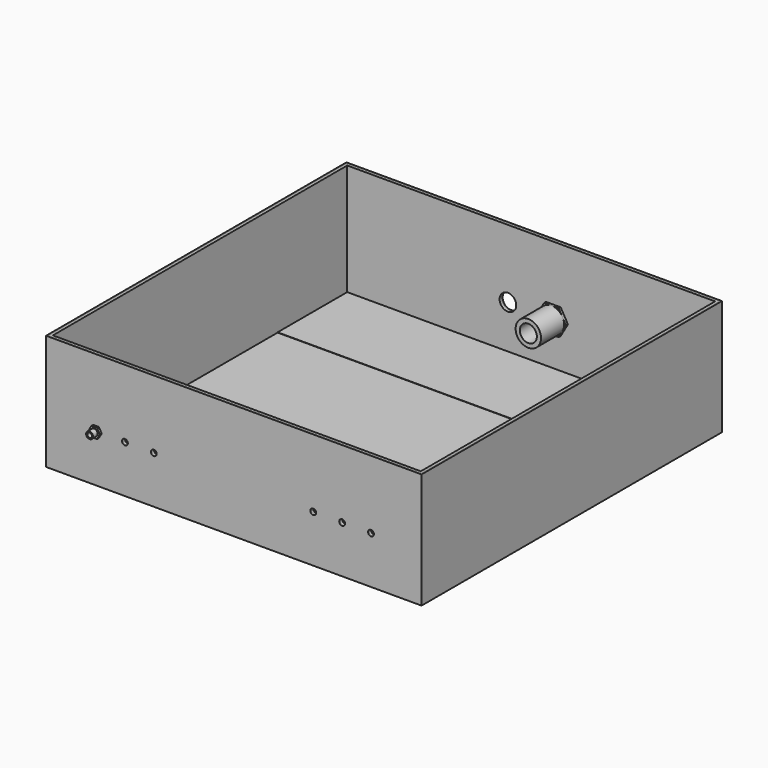
from build123d import *

# Parameters (mm, degrees)
F0_W      = 650
F0_H      = 650
F1_DEPTH  = 200
F2_T      = -2.5
F3_DEPTH  = 197.5
F4_T      = -4
F5_W      = 637
F5_H      = 150.622
F6_DEPTH  = 0.5
F7_R      = 5
F8_DEPTH  = 25
F9_R      = 14.3895
F10_DEPTH = 15
F11_R     = 4
F12_DEPTH = 4
F13_R     = 6
F13_R_2   = 4
F14_DEPTH = 10
F15_R     = 5
F15_R_2   = 4
F16_DEPTH = 6.5
F17_R     = 5
F17_R_2   = 4
F18_DEPTH = 4
F19_R     = 6
F19_R_2   = 5
F20_DEPTH = 150
F21_R     = 11.3895
F22_DEPTH = 4
F23_R     = 13.0309314184
F23_R_2   = 11.3895
F24_DEPTH = 25
F25_R     = 14.3895
F25_R_2   = 11.3895
F26_DEPTH = 6.5
F27_R     = 11.3895
F28_DEPTH = 4
F29_R     = 22.0019443752
F29_R_2   = 14.7554030698
F30_DEPTH = 50


# Not quite as in the source:
# - a feature names something its author has since deleted; it is built from what else it names


with BuildPart() as f1:
    # F0 (on Top) → F1 (new body)
    with BuildSketch(Plane.XY):
        Rectangle(F0_W, F0_H)
    extrude(amount=F1_DEPTH)

    # F2
    f2_openings = [f1.faces().sort_by_distance(p)[0] for p in [
        (0, 0, 200),
    ]]
    offset(amount=F2_T, openings=f2_openings)


with BuildPart() as f3:
    # F3 (new): a face of the model
    f3_faces = [f1.part.faces().sort_by_distance(p)[0] for p in [
        (0, 0, 2.5),
    ]]
    extrude(f3_faces, amount=F3_DEPTH)

    # F4
    f4_openings = [f3.faces().sort_by_distance(p)[0] for p in [
        (0, 0, 200),
    ]]
    offset(amount=F4_T, openings=f4_openings)

    # F5 (on face) → F6 (join)
    with BuildSketch(Plane.XY.offset(6.5)):
        with Locations((0, 243.189)):
            Rectangle(F5_W, F5_H)
    extrude(amount=F6_DEPTH)


with BuildPart() as f8_tool:
    # F7 (on face) → F8 (new body)
    with BuildSketch(Plane.XZ.offset(325)):
        with Locations((-238.5, 82.182)):
            Circle(F7_R)
        with Locations((-188.5, 82.182)):
            Circle(F7_R)
        with Locations((-138.5, 82.182)):
            Circle(F7_R)
        with Locations((237.5, 82.065)):
            Circle(F7_R)
        with Locations((187.5, 82.065)):
            Circle(F7_R)
        with Locations((137.5, 82.065)):
            Circle(F7_R)
    extrude(amount=-F8_DEPTH)


with BuildPart() as f1_1:
    add(f1.part)

    # F8: cut by f8_tool
    add(f8_tool.part, mode=Mode.SUBTRACT)


with BuildPart() as f3_1:
    add(f3.part)

    # F8: cut by f8_tool
    add(f8_tool.part, mode=Mode.SUBTRACT)


with BuildPart() as f10_tool:
    # F9 (on face) → F10 (new body)
    with BuildSketch(Plane(origin=(0, 325, 0), x_dir=(-1, 0, 0), z_dir=(0, 1, 0))):
        with Locations((40.25, 82.065)):
            Circle(F9_R)
        with Locations((-38.25, 82.065)):
            Circle(F9_R)
    extrude(amount=-F10_DEPTH)


with BuildPart() as f1_2:
    add(f1_1.part)

    # F10: cut by f10_tool
    add(f10_tool.part, mode=Mode.SUBTRACT)


with BuildPart() as f3_2:
    add(f3_1.part)

    # F10: cut by f10_tool
    add(f10_tool.part, mode=Mode.SUBTRACT)


with BuildPart() as f12:
    # F11 (on face) → F12 (new body)
    with BuildSketch(Plane.XZ.offset(325)):
        Polygon((-233.5925227119, 90.682), (-243.4074772881, 90.682), (-248.3149545762, 82.182), (-243.4074772881, 73.682), (-233.5925227119, 73.682), (-228.6850454238, 82.182), align=None)
        with Locations((-238.5, 82.182)):
            Circle(F11_R, mode=Mode.SUBTRACT)
    extrude(amount=F12_DEPTH)

    # F13 (on face) → F14 (join)
    with BuildSketch(Plane.XZ.offset(329)):
        with Locations((-238.5, 82.182)):
            Circle(F13_R)
        with Locations((-238.5, 82.182)):
            Circle(F13_R_2, mode=Mode.SUBTRACT)
    extrude(amount=F14_DEPTH)

    # F15 (on face) → F16 (join)
    with BuildSketch(Plane(origin=(0, -325, 0), x_dir=(-1, 0, 0), z_dir=(0, 1, 0))):
        with Locations((238.5, 82.182)):
            Circle(F15_R)
        with Locations((238.5, 82.182)):
            Circle(F15_R_2, mode=Mode.SUBTRACT)
    extrude(amount=F16_DEPTH)

    # F17 (on face) → F18 (join)
    with BuildSketch(Plane(origin=(0, -318.5, 0), x_dir=(-1, 0, 0), z_dir=(0, 1, 0))):
        Polygon((243.4074772881, 90.682), (233.5925227119, 90.682), (228.6850454238, 82.182), (233.5925227119, 73.682), (243.4074772881, 73.682), (248.3149545762, 82.182), align=None)
        with Locations((238.5, 82.182)):
            Circle(F17_R, mode=Mode.SUBTRACT)
        with Locations((238.5, 82.182)):
            Circle(F17_R)
        with Locations((238.5, 82.182)):
            Circle(F17_R_2, mode=Mode.SUBTRACT)
    extrude(amount=F18_DEPTH)

    # F19 (on face) → F20 (join)
    with BuildSketch(Plane(origin=(0, -314.5, 0), x_dir=(-1, 0, 0), z_dir=(0, 1, 0))):
        with Locations((238.5, 82.182)):
            Circle(F19_R)
        with Locations((238.5, 82.182)):
            Circle(F19_R_2, mode=Mode.SUBTRACT)
    extrude(amount=F20_DEPTH)


with BuildPart() as f22:
    # F21 (on face) → F22 (new body)
    with BuildSketch(Plane(origin=(0, 325, 0), x_dir=(-1, 0, 0), z_dir=(0, 1, 0))):
        Polygon((-28.1578817366, 99.5450615883), (-48.3421182634, 99.5450615883), (-58.4342365269, 82.065), (-48.3421182634, 64.5849384117), (-28.1578817366, 64.5849384117), (-18.0657634731, 82.065), align=None)
        with Locations((-38.25, 82.065)):
            Circle(F21_R, mode=Mode.SUBTRACT)
    extrude(amount=F22_DEPTH)

    # F23 (on face) → F24 (join)
    with BuildSketch(Plane(origin=(0, 329, 0), x_dir=(-1, 0, 0), z_dir=(0, 1, 0))):
        with Locations((-38.25, 82.065)):
            Circle(F23_R)
        with Locations((-38.25, 82.065)):
            Circle(F23_R_2, mode=Mode.SUBTRACT)
    extrude(amount=F24_DEPTH)

    # F25 (on face) → F26 (join)
    with BuildSketch(Plane.XZ.offset(-325)):
        with Locations((38.25, 82.065)):
            Circle(F25_R)
        with Locations((38.25, 82.065)):
            Circle(F25_R_2, mode=Mode.SUBTRACT)
    extrude(amount=F26_DEPTH)

    # F27 (on face) → F28 (join)
    with BuildSketch(Plane.XZ.offset(-318.5)):
        Polygon((50.9528285077, 104.0669443752), (25.5471714923, 104.0669443752), (12.8443429845, 82.065), (25.5471714923, 60.0630556248), (50.9528285077, 60.0630556248), (63.6556570155, 82.065), align=None)
        with Locations((38.25, 82.065)):
            Circle(F27_R, mode=Mode.SUBTRACT)
    extrude(amount=F28_DEPTH)

    # F29 (on face) → F30 (join)
    with BuildSketch(Plane.XZ.offset(-314.5)):
        with Locations((38.25, 82.065)):
            Circle(F29_R)
        with Locations((38.25, 82.065)):
            Circle(F29_R_2, mode=Mode.SUBTRACT)
    extrude(amount=F30_DEPTH)


solid = Compound([f1_2.part, f3_2.part, f12.part, f22.part])
